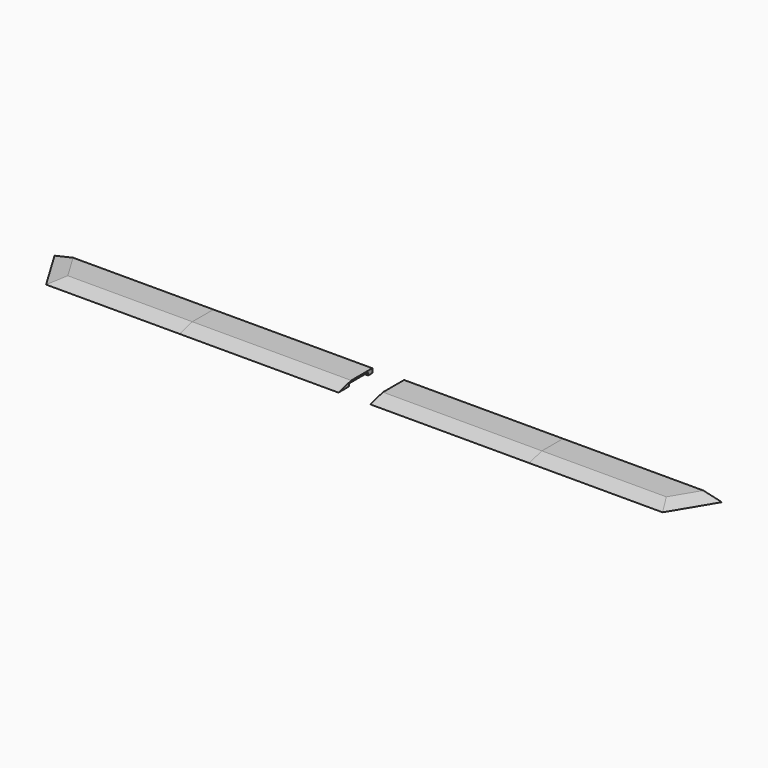
from build123d import *

# Parameters (mm, degrees)
F1_DEPTH   = 4
F0_W       = 150
F0_H       = 40
F2_DEPTH   = 4
F3_SIZE2   = 3.99999
F3_SIZE    = 14.99999
F3_2_SIZE2 = 3.99999
F3_2_SIZE  = 14.99999
F4_SIZE2   = 14.99999
F4_SIZE    = 3.99999
F4_2_SIZE2 = 14.99999
F4_2_SIZE  = 3.99999
F4_3_SIZE2 = 14.99999
F4_3_SIZE  = 3.99999
F5_W       = 100
F5_H       = 22.5
F5_W_2     = 70
F6_DEPTH   = 2.5


# Not quite as in the source:
# - a fillet or chamfer is up to 0.001 mm smaller than in the source, because OpenCascade refuses the exact size


with BuildPart() as f1:
    # F0 (on Top) → F1 (new body)
    with BuildSketch(Plane.XY):
        Polygon((-291, 0), (-165, 0), (-165, 40), (-315, 40), align=None)
    extrude(amount=F1_DEPTH)

    # F4 (size 4 and 15 in the source; OpenCascade refuses exactly that, so slightly less here)
    f4_edges = [f1.edges().sort_by_distance(p)[0] for p in [
        (-228, 0, 4),
        (-303, 20, 4),
    ]]
    chamfer(f4_edges, length=F4_SIZE, length2=F4_SIZE2)


with BuildPart() as f1b:
    # F0 (on Top) → F1, piece 2 (new body)
    with BuildSketch(Plane.XY):
        Polygon((165, 40), (165, 0), (291, 0), (315, 40), align=None)
    extrude(amount=F1_DEPTH)

    # F3#2 (size 15 and 4 in the source; OpenCascade refuses exactly that, so slightly less here)
    f3_2_edges = [f1b.edges().sort_by_distance(p)[0] for p in [
        (303, 20, 4),
    ]]
    f3_2_side = f1b.faces().sort_by_distance((234.173913, 20.57971, 4))[0]
    chamfer(f3_2_edges, length=F3_2_SIZE, length2=F3_2_SIZE2, reference=f3_2_side)

    # F4#3 (size 4 and 15 in the source; OpenCascade refuses exactly that, so slightly less here)
    f4_3_edges = [f1b.edges().sort_by_distance(p)[0] for p in [
        (219.253578, 0, 4),
    ]]
    chamfer(f4_3_edges, length=F4_3_SIZE, length2=F4_3_SIZE2)


with BuildPart() as f2:
    # F0 (on Top) → F2 (new body)
    with BuildSketch(Plane.XY):
        with Locations((-90, 20)):
            Rectangle(F0_W, F0_H)
    extrude(amount=F2_DEPTH)

    # F4#2 (size 4 and 15 in the source; OpenCascade refuses exactly that, so slightly less here)
    f4_2_edges = [f2.edges().sort_by_distance(p)[0] for p in [
        (-90, 0, 4),
    ]]
    chamfer(f4_2_edges, length=F4_2_SIZE, length2=F4_2_SIZE2)


with BuildPart() as f2b:
    # F0 (on Top) → F2, piece 2 (new body)
    with BuildSketch(Plane.XY):
        with Locations((90, 20)):
            Rectangle(F0_W, F0_H)
    extrude(amount=F2_DEPTH)

    # F3 (size 15 and 4 in the source; OpenCascade refuses exactly that, so slightly less here)
    f3_edges = [f2b.edges().sort_by_distance(p)[0] for p in [
        (90, 0, 4),
    ]]
    f3_side = f2b.faces().sort_by_distance((90, 20, 4))[0]
    chamfer(f3_edges, length=F3_SIZE, length2=F3_SIZE2, reference=f3_side)


with BuildPart() as f6_tool:
    # F5 (on face) → F6 (new body)
    with BuildSketch(Plane.XY):
        with Locations((165, 23.75)):
            Rectangle(F5_W, F5_H)
        with Locations((50, 23.75)):
            Rectangle(F5_W_2, F5_H)
        with Locations((-165, 23.75)):
            Rectangle(F5_W, F5_H)
        with Locations((-50, 23.75)):
            Rectangle(F5_W_2, F5_H)
    extrude(amount=F6_DEPTH)


with BuildPart() as f1_1:
    add(f1.part)

    # F6: cut by f6_tool
    add(f6_tool.part, mode=Mode.SUBTRACT)


with BuildPart() as f1b_1:
    add(f1b.part)

    # F6: cut by f6_tool
    add(f6_tool.part, mode=Mode.SUBTRACT)


with BuildPart() as f2_1:
    add(f2.part)

    # F6: cut by f6_tool
    add(f6_tool.part, mode=Mode.SUBTRACT)


with BuildPart() as f2b_1:
    add(f2b.part)

    # F6: cut by f6_tool
    add(f6_tool.part, mode=Mode.SUBTRACT)


solid = Compound([f1_1.part, f1b_1.part, f2_1.part, f2b_1.part])
